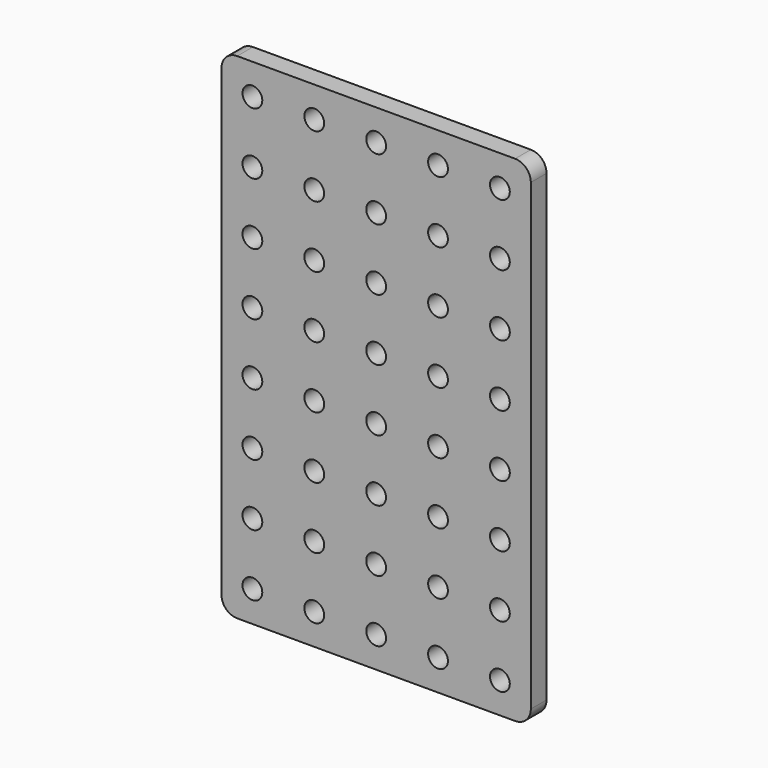
from build123d import *

# Parameters (mm, degrees)
F0_R     = 1.6
F1_DEPTH = 3.175


# Not quite as in the source:
# - a length typed as a fraction of an inch, garbled in the dataset ("3 / 203.2 mm" for 3/8 in), is restored


with BuildPart() as f1:
    # F0 (on Front) → F1 (new body)
    with BuildSketch(Plane.XZ):
        with BuildLine():
            Line((47.46, 0), (2.54, 0))
            ThreePointArc((2.54, 0), (0.7439487758, -0.7439487758), (0, -2.54))
            Line((0, -2.54), (0, -77.46))
            ThreePointArc((0, -77.46), (0.7439487758, -79.2560512242), (2.54, -80))
            Line((2.54, -80), (47.46, -80))
            ThreePointArc((47.46, -80), (49.2560512242, -79.2560512242), (50, -77.46))
            Line((50, -77.46), (50, -2.54))
            ThreePointArc((50, -2.54), (49.2560512242, -0.7439487758), (47.46, 0))
        make_face()
        with Locations((5, -75)):
            Circle(F0_R, mode=Mode.SUBTRACT)
        with Locations((5, -65)):
            Circle(F0_R, mode=Mode.SUBTRACT)
        with Locations((15, -75)):
            Circle(F0_R, mode=Mode.SUBTRACT)
        with Locations((15, -65)):
            Circle(F0_R, mode=Mode.SUBTRACT)
        with Locations((5, -55)):
            Circle(F0_R, mode=Mode.SUBTRACT)
        with Locations((5, -45)):
            Circle(F0_R, mode=Mode.SUBTRACT)
        with Locations((15, -55)):
            Circle(F0_R, mode=Mode.SUBTRACT)
        with Locations((15, -45)):
            Circle(F0_R, mode=Mode.SUBTRACT)
        with Locations((25, -75)):
            Circle(F0_R, mode=Mode.SUBTRACT)
        with Locations((35, -75)):
            Circle(F0_R, mode=Mode.SUBTRACT)
        with Locations((25, -65)):
            Circle(F0_R, mode=Mode.SUBTRACT)
        with Locations((35, -65)):
            Circle(F0_R, mode=Mode.SUBTRACT)
        with Locations((45, -75)):
            Circle(F0_R, mode=Mode.SUBTRACT)
        with Locations((45, -65)):
            Circle(F0_R, mode=Mode.SUBTRACT)
        with Locations((25, -55)):
            Circle(F0_R, mode=Mode.SUBTRACT)
        with Locations((35, -55)):
            Circle(F0_R, mode=Mode.SUBTRACT)
        with Locations((25, -45)):
            Circle(F0_R, mode=Mode.SUBTRACT)
        with Locations((35, -45)):
            Circle(F0_R, mode=Mode.SUBTRACT)
        with Locations((45, -55)):
            Circle(F0_R, mode=Mode.SUBTRACT)
        with Locations((45, -45)):
            Circle(F0_R, mode=Mode.SUBTRACT)
        with Locations((5, -35)):
            Circle(F0_R, mode=Mode.SUBTRACT)
        with Locations((5, -25)):
            Circle(F0_R, mode=Mode.SUBTRACT)
        with Locations((15, -35)):
            Circle(F0_R, mode=Mode.SUBTRACT)
        with Locations((15, -25)):
            Circle(F0_R, mode=Mode.SUBTRACT)
        with Locations((5, -15)):
            Circle(F0_R, mode=Mode.SUBTRACT)
        with Locations((5, -5)):
            Circle(F0_R, mode=Mode.SUBTRACT)
        with Locations((15, -15)):
            Circle(F0_R, mode=Mode.SUBTRACT)
        with Locations((15, -5)):
            Circle(F0_R, mode=Mode.SUBTRACT)
        with Locations((25, -35)):
            Circle(F0_R, mode=Mode.SUBTRACT)
        with Locations((35, -35)):
            Circle(F0_R, mode=Mode.SUBTRACT)
        with Locations((25, -25)):
            Circle(F0_R, mode=Mode.SUBTRACT)
        with Locations((35, -25)):
            Circle(F0_R, mode=Mode.SUBTRACT)
        with Locations((45, -35)):
            Circle(F0_R, mode=Mode.SUBTRACT)
        with Locations((45, -25)):
            Circle(F0_R, mode=Mode.SUBTRACT)
        with Locations((25, -15)):
            Circle(F0_R, mode=Mode.SUBTRACT)
        with Locations((35, -15)):
            Circle(F0_R, mode=Mode.SUBTRACT)
        with Locations((25, -5)):
            Circle(F0_R, mode=Mode.SUBTRACT)
        with Locations((35, -5)):
            Circle(F0_R, mode=Mode.SUBTRACT)
        with Locations((45, -15)):
            Circle(F0_R, mode=Mode.SUBTRACT)
        with Locations((45, -5)):
            Circle(F0_R, mode=Mode.SUBTRACT)
    extrude(amount=F1_DEPTH)


solid = f1.part
